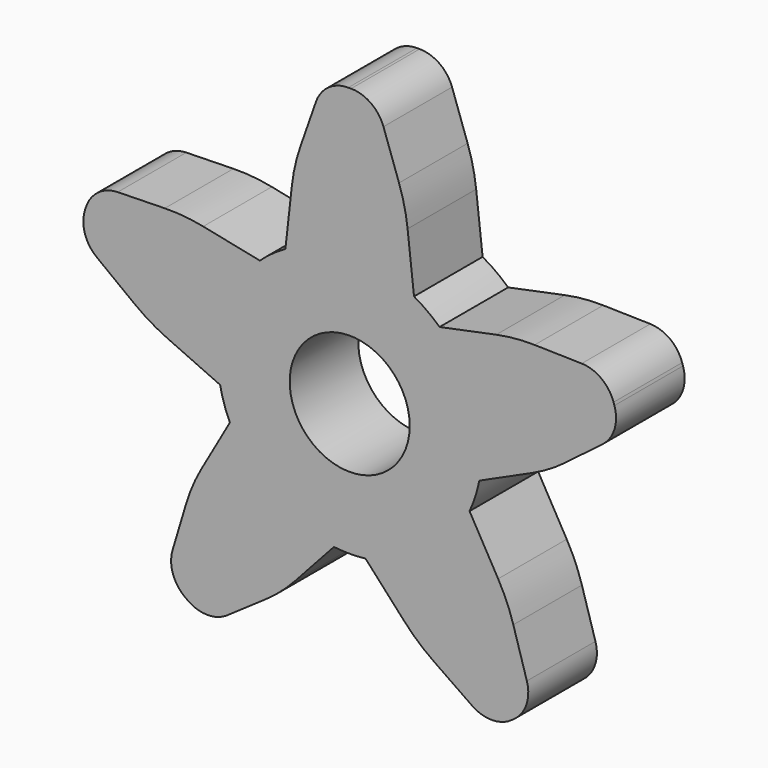
from build123d import *

# Parameters (mm, degrees)
F0_R     = 1.778
F1_DEPTH = 2.54
F2_R     = 5.08
F3_R     = 1.016


# Not quite as in the source:
# - a feature names something its author has since deleted; it is built from what else it names


with BuildPart() as f1:
    # F0 (on Front) → F1 (new body)
    with BuildSketch(Plane.XZ):
        with BuildLine():
            Line((0.762, 12.192), (-0.762, 12.192))
            Line((-0.762, 12.192), (-1.651, 9.652))
            Line((-1.651, 9.652), (-1.905, 7.3780332745))
            ThreePointArc((-1.905, 7.3780332745), (0, 7.8729912016), (1.905, 7.3780332745))
            Line((1.905, 7.3780332745), (1.651, 9.652))
            Line((1.651, 9.652), (0.762, 12.192))
        make_face()
        with BuildLine():
            ThreePointArc((1.905, 7.3780332745), (0, 7.8729912016), (-1.905, 7.3780332745))
            ThreePointArc((-1.905, 7.3780332745), (-2.3002813477, 7.1255844849), (-2.6625230681, 6.8276605496))
            ThreePointArc((-2.6625230681, 6.8276605496), (-3.7219334042, 5.168848297), (-3.8398778167, 3.2041352225))
            ThreePointArc((-3.8398778167, 3.2041352225), (-3.7219334042, 2.7501893548), (-3.5505297519, 2.3136134471))
            ThreePointArc((-3.5505297519, 2.3136134471), (-2.3002813477, 0.793453167), (-0.4681750033, 0.0741516359))
            ThreePointArc((-0.4681750033, 0.0741516359), (0, 0.0460464502), (0.4681750033, 0.0741516359))
            ThreePointArc((0.4681750033, 0.0741516359), (2.3002813477, 0.793453167), (3.5505297519, 2.3136134471))
            ThreePointArc((3.5505297519, 2.3136134471), (3.7219334042, 2.7501893548), (3.8398778167, 3.2041352225))
            ThreePointArc((3.8398778167, 3.2041352225), (3.8950302821, 3.5800387384), (3.9134723757, 3.9595188259))
            ThreePointArc((3.9134723757, 3.9595188259), (3.5871281349, 5.5240563868), (2.6625230681, 6.8276605496))
            ThreePointArc((2.6625230681, 6.8276605496), (2.3002813477, 7.1255844849), (1.905, 7.3780332745))
        make_face()
        with Locations((0, 3.9595188259)):
            Circle(F0_R, mode=Mode.SUBTRACT)
        with BuildLine():
            ThreePointArc((-3.8398778167, 3.2041352225), (-3.7219334042, 5.168848297), (-2.6625230681, 6.8276605496))
            Line((-2.6625230681, 6.8276605496), (-4.9036842568, 7.2887865573))
            Line((-4.9036842568, 7.2887865573), (-7.5940839162, 7.22820048))
            Line((-7.5940839162, 7.22820048), (-8.0650258156, 5.7787903492))
            Line((-8.0650258156, 5.7787903492), (-5.9240583722, 4.1483979405))
            Line((-5.9240583722, 4.1483979405), (-3.8398778167, 3.2041352225))
        make_face()
        with BuildLine():
            Line((4.9036842568, 7.2887865573), (2.6625230681, 6.8276605496))
            ThreePointArc((2.6625230681, 6.8276605496), (3.5871281349, 5.5240563868), (3.9134723757, 3.9595188259))
            ThreePointArc((3.9134723757, 3.9595188259), (3.8950302821, 3.5800387384), (3.8398778167, 3.2041352225))
            Line((3.8398778167, 3.2041352225), (5.9240583722, 4.1483979405))
            Line((5.9240583722, 4.1483979405), (8.0650258156, 5.7787903492))
            Line((8.0650258156, 5.7787903492), (7.5940839162, 7.22820048))
            Line((7.5940839162, 7.22820048), (4.9036842568, 7.2887865573))
        make_face()
        with BuildLine():
            ThreePointArc((-0.4681750033, 0.0741516359), (-2.3002813477, 0.793453167), (-3.5505297519, 2.3136134471))
            Line((-3.5505297519, 2.3136134471), (-4.6816435408, 0.3246382675))
            Line((-4.6816435408, 0.3246382675), (-5.4554019736, -2.2528059875))
            Line((-5.4554019736, -2.2528059875), (-4.2224600742, -3.148590712))
            Line((-4.2224600742, -3.148590712), (-2.0102694254, -1.6162286356))
            Line((-2.0102694254, -1.6162286356), (-0.4681750033, 0.0741516359))
        make_face()
        with BuildLine():
            Line((4.6816435408, 0.3246382675), (3.5505297519, 2.3136134471))
            ThreePointArc((3.5505297519, 2.3136134471), (2.3002813477, 0.793453167), (0.4681750033, 0.0741516359))
            Line((0.4681750033, 0.0741516359), (2.0102694254, -1.6162286356))
            Line((2.0102694254, -1.6162286356), (4.2224600742, -3.148590712))
            Line((4.2224600742, -3.148590712), (5.4554019736, -2.2528059875))
            Line((5.4554019736, -2.2528059875), (4.6816435408, 0.3246382675))
        make_face()
    extrude(amount=F1_DEPTH)

    # F2
    f2_edges = [f1.edges().sort_by_distance(p)[0] for p in [
        (1.651, -1.27, 9.652),
        (-4.903684, -1.27, 7.288787),
        (-4.681644, -1.27, 0.324638),
        (2.010269, -1.27, -1.616229),
        (5.924058, -1.27, 4.148398),
        (-1.651, -1.27, 9.652),
        (-5.924058, -1.27, 4.148398),
        (-2.010269, -1.27, -1.616229),
        (4.681644, -1.27, 0.324638),
        (4.903684, -1.27, 7.288787),
    ]]
    fillet(f2_edges, radius=F2_R)

    # F3
    f3_edges = [f1.edges().sort_by_distance(p)[0] for p in [
        (0.762, -1.27, 12.192),
        (-0.762, -1.27, 12.192),
        (-7.594084, -1.27, 7.2282),
        (-8.065026, -1.27, 5.77879),
        (-5.455402, -1.27, -2.252806),
        (-4.22246, -1.27, -3.148591),
        (4.22246, -1.27, -3.148591),
        (5.455402, -1.27, -2.252806),
        (8.065026, -1.27, 5.77879),
        (7.594084, -1.27, 7.2282),
    ]]
    fillet(f3_edges, radius=F3_R)


solid = f1.part
